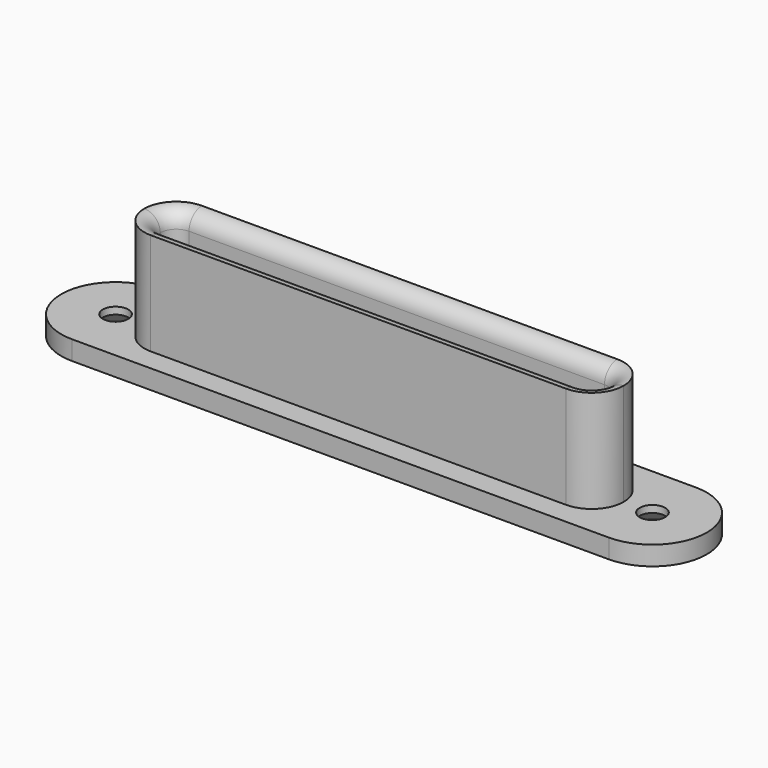
from build123d import *

# Parameters (mm, degrees)
F0_R     = 4
F0_R_2   = 2
F1_DEPTH = 2
F2_DEPTH = 1
F3_DEPTH = 2.001
F4_DEPTH = 18
F5_DEPTH = 18.001
F6_R     = 2.49999
F7_SIZE  = 1.9


# Not quite as in the source:
# - a fillet or chamfer is up to 0.001 mm smaller than in the source, because OpenCascade refuses the exact size


with BuildPart() as f1:
    # F0 (on Top) → F1 (new body)
    with BuildSketch(Plane.XY):
        with BuildLine():
            ThreePointArc((42, -8.5), (50.5, 0), (42, 8.5))
            Line((42, 8.5), (-42, 8.5))
            ThreePointArc((-42, 8.5), (-50.5, 0), (-42, -8.5))
            Line((-42, -8.5), (42, -8.5))
        make_face()
        with BuildLine():
            ThreePointArc((37.5, 0), (36.035534, -3.535534), (32.5, -5))
            Line((32.5, -5), (-32.5, -5))
            ThreePointArc((-32.5, -5), (-36.035534, -3.535534), (-37.5, 0))
            ThreePointArc((-37.5, 0), (-36.035534, 3.535534), (-32.5, 5))
            Line((-32.5, 5), (32.5, 5))
            ThreePointArc((32.5, 5), (36.035534, 3.535534), (37.5, 0))
        make_face(mode=Mode.SUBTRACT)
        with Locations((-42, 0)):
            Circle(F0_R, mode=Mode.SUBTRACT)
        with Locations((42, 0)):
            Circle(F0_R, mode=Mode.SUBTRACT)
        with BuildLine():
            Line((-32.5, -5), (32.5, -5))
            ThreePointArc((32.5, -5), (36.035534, -3.535534), (37.5, 0))
            ThreePointArc((37.5, 0), (36.035534, 3.535534), (32.5, 5))
            Line((32.5, 5), (-32.5, 5))
            ThreePointArc((-32.5, 5), (-36.035534, 3.535534), (-37.5, 0))
            ThreePointArc((-37.5, 0), (-36.035534, -3.535534), (-32.5, -5))
        make_face()
        with BuildLine():
            ThreePointArc((35, 0), (34.267767, -1.767767), (32.5, -2.5))
            Line((32.5, -2.5), (-32.5, -2.5))
            ThreePointArc((-32.5, -2.5), (-34.267767, -1.767767), (-35, 0))
            ThreePointArc((-35, 0), (-34.267767, 1.767767), (-32.5, 2.5))
            Line((-32.5, 2.5), (32.5, 2.5))
            ThreePointArc((32.5, 2.5), (34.267767, 1.767767), (35, 0))
        make_face(mode=Mode.SUBTRACT)
        with BuildLine():
            Line((-32.5, -2.5), (32.5, -2.5))
            ThreePointArc((32.5, -2.5), (34.267767, -1.767767), (35, 0))
            ThreePointArc((35, 0), (34.267767, 1.767767), (32.5, 2.5))
            Line((32.5, 2.5), (-32.5, 2.5))
            ThreePointArc((-32.5, 2.5), (-34.267767, 1.767767), (-35, 0))
            ThreePointArc((-35, 0), (-34.267767, -1.767767), (-32.5, -2.5))
        make_face()
        with Locations((42, 0)):
            Circle(F0_R)
        with Locations((42, 0)):
            Circle(F0_R_2, mode=Mode.SUBTRACT)
        with Locations((-42, 0)):
            Circle(F0_R)
        with Locations((-42, 0)):
            Circle(F0_R_2, mode=Mode.SUBTRACT)
        with Locations((-42, 0)):
            Circle(F0_R_2)
        with Locations((42, 0)):
            Circle(F0_R_2)
    extrude(amount=F1_DEPTH)

    # F0 (on Top) → F2 (join)
    with BuildSketch(Plane.XY):
        with BuildLine():
            ThreePointArc((42, -8.5), (50.5, 0), (42, 8.5))
            Line((42, 8.5), (-42, 8.5))
            ThreePointArc((-42, 8.5), (-50.5, 0), (-42, -8.5))
            Line((-42, -8.5), (42, -8.5))
        make_face()
        with BuildLine():
            ThreePointArc((37.5, 0), (36.035534, -3.535534), (32.5, -5))
            Line((32.5, -5), (-32.5, -5))
            ThreePointArc((-32.5, -5), (-36.035534, -3.535534), (-37.5, 0))
            ThreePointArc((-37.5, 0), (-36.035534, 3.535534), (-32.5, 5))
            Line((-32.5, 5), (32.5, 5))
            ThreePointArc((32.5, 5), (36.035534, 3.535534), (37.5, 0))
        make_face(mode=Mode.SUBTRACT)
        with Locations((-42, 0)):
            Circle(F0_R, mode=Mode.SUBTRACT)
        with Locations((42, 0)):
            Circle(F0_R, mode=Mode.SUBTRACT)
        with BuildLine():
            Line((-32.5, -5), (32.5, -5))
            ThreePointArc((32.5, -5), (36.035534, -3.535534), (37.5, 0))
            ThreePointArc((37.5, 0), (36.035534, 3.535534), (32.5, 5))
            Line((32.5, 5), (-32.5, 5))
            ThreePointArc((-32.5, 5), (-36.035534, 3.535534), (-37.5, 0))
            ThreePointArc((-37.5, 0), (-36.035534, -3.535534), (-32.5, -5))
        make_face()
        with BuildLine():
            ThreePointArc((35, 0), (34.267767, -1.767767), (32.5, -2.5))
            Line((32.5, -2.5), (-32.5, -2.5))
            ThreePointArc((-32.5, -2.5), (-34.267767, -1.767767), (-35, 0))
            ThreePointArc((-35, 0), (-34.267767, 1.767767), (-32.5, 2.5))
            Line((-32.5, 2.5), (32.5, 2.5))
            ThreePointArc((32.5, 2.5), (34.267767, 1.767767), (35, 0))
        make_face(mode=Mode.SUBTRACT)
        with Locations((-42, 0)):
            Circle(F0_R)
        with Locations((-42, 0)):
            Circle(F0_R_2, mode=Mode.SUBTRACT)
        with Locations((42, 0)):
            Circle(F0_R)
        with Locations((42, 0)):
            Circle(F0_R_2, mode=Mode.SUBTRACT)
    extrude(amount=-F2_DEPTH)

    # F0 (on Top) → F3 (cut, through all)
    with BuildSketch(Plane.XY):
        with Locations((42, 0)):
            Circle(F0_R_2)
        with Locations((-42, 0)):
            Circle(F0_R_2)
    extrude(amount=F3_DEPTH, mode=Mode.SUBTRACT)

    # F0 (on Top) → F4 (join)
    with BuildSketch(Plane.XY):
        with BuildLine():
            Line((-32.5, -5), (32.5, -5))
            ThreePointArc((32.5, -5), (36.035534, -3.535534), (37.5, 0))
            ThreePointArc((37.5, 0), (36.035534, 3.535534), (32.5, 5))
            Line((32.5, 5), (-32.5, 5))
            ThreePointArc((-32.5, 5), (-36.035534, 3.535534), (-37.5, 0))
            ThreePointArc((-37.5, 0), (-36.035534, -3.535534), (-32.5, -5))
        make_face()
        with BuildLine():
            ThreePointArc((35, 0), (34.267767, -1.767767), (32.5, -2.5))
            Line((32.5, -2.5), (-32.5, -2.5))
            ThreePointArc((-32.5, -2.5), (-34.267767, -1.767767), (-35, 0))
            ThreePointArc((-35, 0), (-34.267767, 1.767767), (-32.5, 2.5))
            Line((-32.5, 2.5), (32.5, 2.5))
            ThreePointArc((32.5, 2.5), (34.267767, 1.767767), (35, 0))
        make_face(mode=Mode.SUBTRACT)
    extrude(amount=F4_DEPTH)

    # F0 (on Top) → F5 (cut, through all)
    with BuildSketch(Plane.XY):
        with BuildLine():
            Line((-32.5, -2.5), (32.5, -2.5))
            ThreePointArc((32.5, -2.5), (34.267767, -1.767767), (35, 0))
            ThreePointArc((35, 0), (34.267767, 1.767767), (32.5, 2.5))
            Line((32.5, 2.5), (-32.5, 2.5))
            ThreePointArc((-32.5, 2.5), (-34.267767, 1.767767), (-35, 0))
            ThreePointArc((-35, 0), (-34.267767, -1.767767), (-32.5, -2.5))
        make_face()
    extrude(amount=F5_DEPTH, mode=Mode.SUBTRACT)

    # F6 (radius 2.5 in the source; OpenCascade refuses exactly that, so slightly less here)
    f6_edges = [f1.edges().sort_by_distance(p)[0] for p in [
        (0, 2.5, -1),
        (0, -2.5, 18),
    ]]
    fillet(f6_edges, radius=F6_R)

    # F7
    f7_edges = [f1.edges().sort_by_distance(p)[0] for p in [
        (-44, 0, -1),
        (40, 0, -1),
    ]]
    chamfer(f7_edges, length=F7_SIZE)


solid = f1.part
